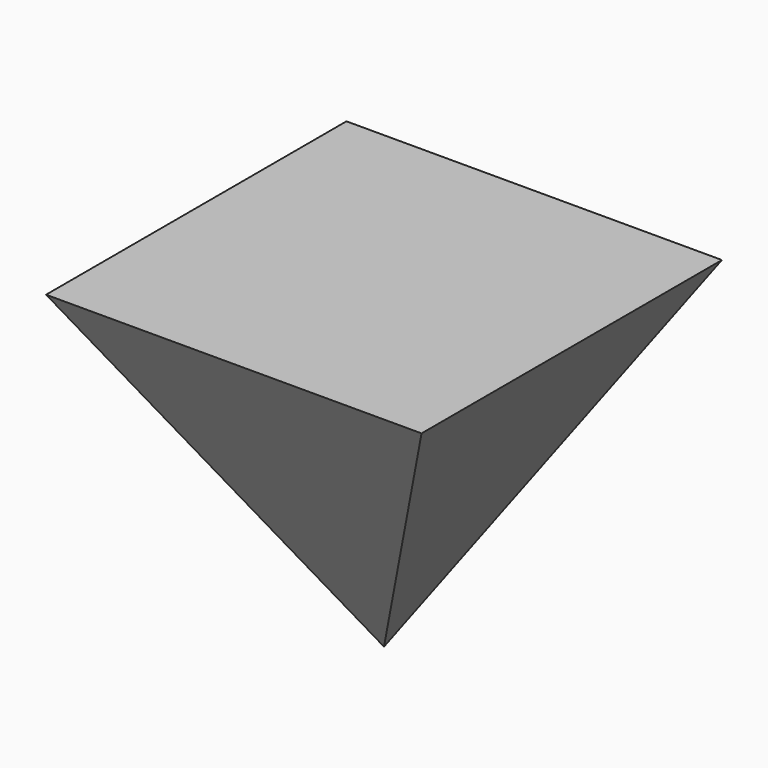
from build123d import *

# Parameters (mm, degrees)
F0_W = 76.2
F0_H = 76.2


# Not quite as in the source:
# - an extrude whose draft closes it to a point is written as a loft to that point


with BuildPart() as f1:
    # F0 (on Top) → F1 section 0
    with BuildSketch(Plane.XY, mode=Mode.PRIVATE) as f1_s0:
        with Locations((-34.3464494912, -38.8499209657)):
            Rectangle(F0_W, F0_H)
    loft([f1_s0.sketch, Vertex(-34.3464494912, -38.8499209657, -65.9911357684)], ruled=True)


solid = f1.part
